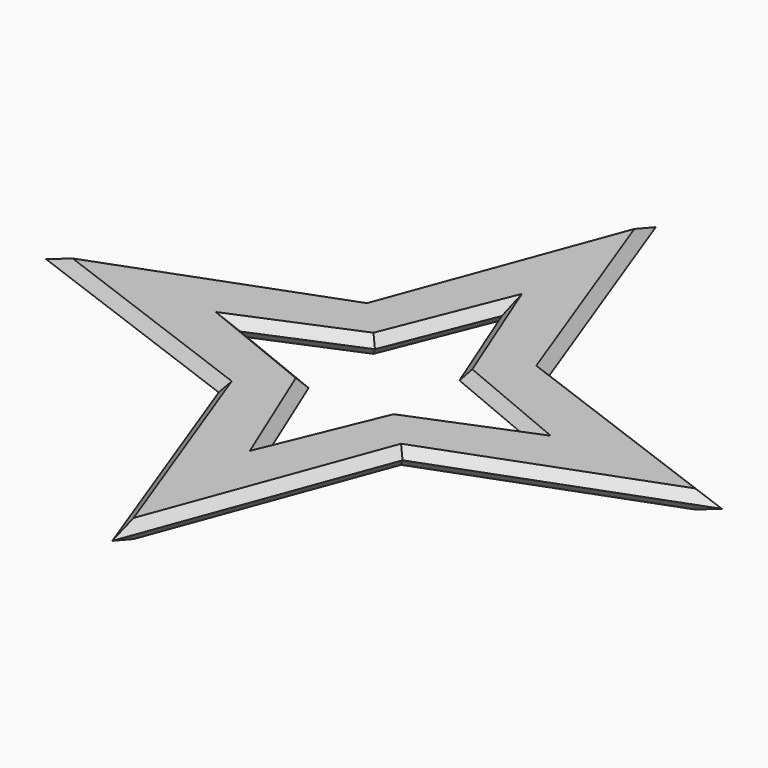
from build123d import *

# Parameters (mm, degrees)
F2_DEPTH = 2.54
F3_DEPTH = 23.622
F4_SIZE  = 1.26999


# Not quite as in the source:
# - a fillet or chamfer is up to 0.001 mm smaller than in the source, because OpenCascade refuses the exact size


with BuildPart() as f2:
    # F0 (on Top) → F2 (new body)
    with BuildSketch(Plane.XY):
        Polygon((12.5471574406, 12.5223604022), (0, 46.3847853243), (-12.5471574406, 12.5223604022), (-46.1385440799, 0), (-12.5471574406, -12.5223604022), (0, -46.3847853243), (12.5471574406, -12.5223604022), (46.1385440799, 0), align=None)
    extrude(amount=F2_DEPTH)

    # F1 (on Top) → F3 (cut)
    with BuildSketch(Plane.XY):
        Polygon((5.7690664033, 5.6696828615), (0, 20.1142430305), (-5.7690664033, 5.6696828615), (-19.5389121215, -0.109308556), (-5.705270301, -5.7338749296), (0, -19.5673167638), (5.705270301, -5.7338749296), (19.5389121215, -0.109308556), align=None)
    extrude(amount=F3_DEPTH, mode=Mode.SUBTRACT)

    # F4 (size 1.27 in the source; OpenCascade refuses exactly that, so slightly less here)
    f4_edges = [f2.edges().sort_by_distance(p)[0] for p in [
        (6.273579, -29.453573, 2.54),
        (-6.273579, -29.453573, 2.54),
        (-29.342851, -6.26118, 2.54),
        (-29.342851, 6.26118, 2.54),
        (-6.273579, 29.453573, 2.54),
        (6.273579, 29.453573, 2.54),
        (29.342851, 6.26118, 2.54),
        (29.342851, -6.26118, 2.54),
        (-6.273579, 29.453573, 0),
        (29.342851, 6.26118, 0),
        (6.273579, 29.453573, 0),
        (29.342851, -6.26118, 0),
        (6.273579, -29.453573, 0),
        (-6.273579, -29.453573, 0),
        (-29.342851, -6.26118, 0),
        (-29.342851, 6.26118, 0),
        (-12.653989, 2.780187, 0),
        (12.653989, 2.780187, 2.54),
        (2.884533, 12.891963, 2.54),
        (-2.884533, 12.891963, 2.54),
        (-12.653989, 2.780187, 2.54),
        (-12.622091, -2.921592, 2.54),
        (-2.852635, -12.650596, 2.54),
        (2.852635, -12.650596, 2.54),
        (12.622091, -2.921592, 2.54),
        (-12.622091, -2.921592, 0),
        (-2.852635, -12.650596, 0),
        (2.852635, -12.650596, 0),
        (12.622091, -2.921592, 0),
        (12.653989, 2.780187, 0),
        (2.884533, 12.891963, 0),
        (-2.884533, 12.891963, 0),
    ]]
    chamfer(f4_edges, length=F4_SIZE)


solid = f2.part
